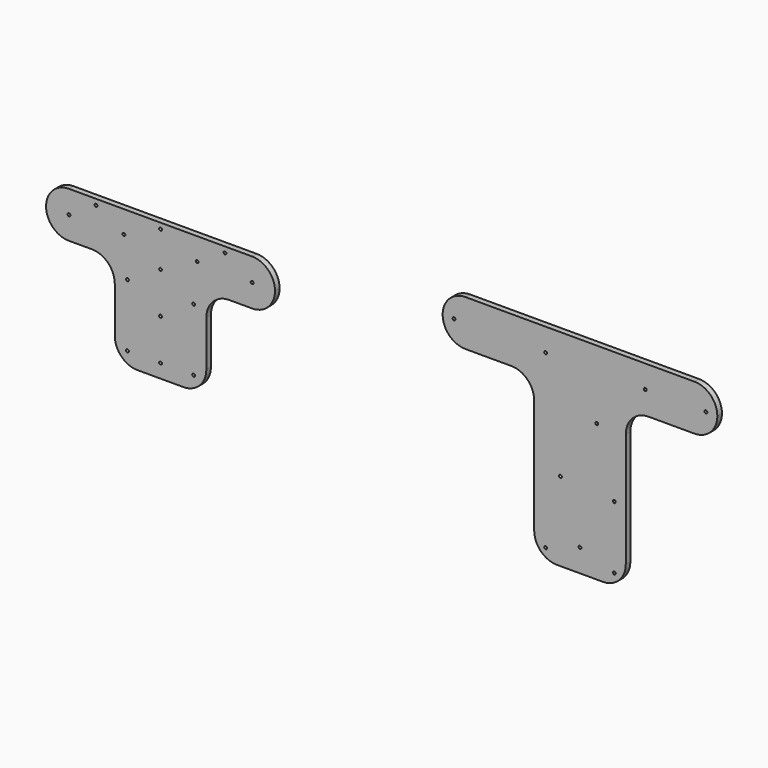
from build123d import *

# Parameters (mm, degrees)
F0_R     = 1.5875
F1_DEPTH = 6.35
F2_R     = 25.39999
F3_R     = 25.4
F4_R     = 25.39999
F5_R     = 1.5875
F6_DEPTH = 25.4


# Not quite as in the source:
# - a fillet or chamfer is up to 0.001 mm smaller than in the source, because OpenCascade refuses the exact size


with BuildPart() as f1:
    # F0 (on Front) → F1 (new body)
    with BuildSketch(Plane.XZ):
        Polygon((50.8, 114.3), (-50.8, 114.3), (-50.8, 63.5), (-50.8, -114.3), (-38.1, -114.3), (38.1, -114.3), (50.8, -114.3), (50.8, -31.75), (50.8, 63.5), (50.8, 88.9428858587), align=None)
        with BuildLine():
            ThreePointArc((-36.5125, -101.6), (-36.9774679849, -102.7225320151), (-38.1, -103.1875))
            ThreePointArc((-38.1, -103.1875), (-39.2225320151, -100.4774679849), (-36.5125, -101.6))
        make_face(mode=Mode.SUBTRACT)
        with BuildLine():
            ThreePointArc((39.6875, -101.6), (39.2225320151, -102.7225320151), (38.1, -103.1875))
            ThreePointArc((38.1, -103.1875), (36.9774679849, -100.4774679849), (39.6875, -101.6))
        make_face(mode=Mode.SUBTRACT)
        with Locations((0, -88.9)):
            Circle(F0_R, mode=Mode.SUBTRACT)
        with Locations((38.1, -31.75)):
            Circle(F0_R, mode=Mode.SUBTRACT)
        with Locations((-21.7083130796, -26.5298890234)):
            Circle(F0_R, mode=Mode.SUBTRACT)
        with Locations((18.6577301353, 38.1)):
            Circle(F0_R, mode=Mode.SUBTRACT)
        with Locations((-38.1000090512, 88.9428858587)):
            Circle(F0_R, mode=Mode.SUBTRACT)
        Polygon((-50.8, 63.5), (-50.8, 114.3), (-152.4, 114.3), (-152.4, 88.9), (-152.4, 63.5), align=None)
        with BuildLine():
            ThreePointArc((-138.1125, 88.9), (-139.7, 87.3125), (-141.2875, 88.9))
            ThreePointArc((-141.2875, 88.9), (-139.7, 90.4875), (-138.1125, 88.9))
        make_face(mode=Mode.SUBTRACT)
        with BuildLine():
            Line((72.3543986678, 114.3), (50.8, 114.3))
            Line((50.8, 114.3), (50.8, 88.9428858587))
            Line((50.8, 88.9428858587), (70.7668986678, 88.9428858587))
            ThreePointArc((70.7668986678, 88.9428858587), (71.2318666527, 90.0654178738), (72.3543986678, 90.5303858587))
            Line((72.3543986678, 90.5303858587), (72.3543986678, 114.3))
        make_face()
        with BuildLine():
            Line((70.7668986678, 88.9428858587), (50.8, 88.9428858587))
            Line((50.8, 88.9428858587), (50.8, 63.5))
            Line((50.8, 63.5), (152.4, 63.5))
            Line((152.4, 63.5), (152.4, 88.9))
            Line((152.4, 88.9), (152.4, 114.3))
            Line((152.4, 114.3), (72.3543986678, 114.3))
            Line((72.3543986678, 114.3), (72.3543986678, 90.5303858587))
            ThreePointArc((72.3543986678, 90.5303858587), (73.4769306829, 90.0654178738), (73.9418986678, 88.9428858587))
            ThreePointArc((73.9418986678, 88.9428858587), (72.3543986678, 87.3553858587), (70.7668986678, 88.9428858587))
        make_face()
        with Locations((139.7, 88.9)):
            Circle(F0_R, mode=Mode.SUBTRACT)
    extrude(amount=F1_DEPTH)

    # F2 (radius 25.4 in the source; OpenCascade refuses exactly that, so slightly less here)
    f2_edges = [f1.edges().sort_by_distance(p)[0] for p in [
        (-50.8, -3.175, 63.5),
        (50.8, -3.175, 63.5),
        (152.4, -3.175, 63.5),
        (152.4, -3.175, 114.3),
        (50.8, -3.175, -114.3),
        (-50.8, -3.175, -114.3),
        (-152.4, -3.175, 63.5),
        (-152.4, -3.175, 114.3),
    ]]
    fillet(f2_edges, radius=F2_R)


with BuildPart() as f1b:
    # F0 (on Front) → F1, piece 2 (new body)
    with BuildSketch(Plane.XZ):
        Polygon((-516.2082994461, 26.1577678084), (-516.2082994461, -75.4422321916), (-414.6082994461, -75.4422321916), (-414.6082994461, 26.1577678084), (-338.4082994461, 26.1577678084), (-338.4082994461, 76.9577678084), (-592.4082994461, 76.9577678084), (-592.4082994461, 26.1577678084), align=None)
        with Locations((-465.4082994461, -60.2022321916)):
            Circle(F0_R, mode=Mode.SUBTRACT)
    extrude(amount=F1_DEPTH)

    # F3
    f3_edges = [f1b.edges().sort_by_distance(p)[0] for p in [
        (-592.408299, -3.175, 26.157768),
        (-516.208299, -3.175, 26.157768),
        (-516.208299, -3.175, -75.442232),
        (-414.608299, -3.175, 26.157768),
        (-414.608299, -3.175, -75.442232),
        (-338.408299, -3.175, 76.957768),
    ]]
    fillet(f3_edges, radius=F3_R)

    # F4 (radius 25.4 in the source; OpenCascade refuses exactly that, so slightly less here)
    f4_edges = [f1b.edges().sort_by_distance(p)[0] for p in [
        (-338.408299, -3.175, 26.157768),
        (-592.408299, -3.175, 76.957768),
    ]]
    fillet(f4_edges, radius=F4_R)

    # F5 (on face) → F6 (cut)
    with BuildSketch(Plane.XZ.offset(6.35)):
        with Locations((-567.0082994461, 51.5577678084)):
            Circle(F5_R)
        with Locations((-363.8082994461, 104.2201220989)):
            Circle(F5_R)
        with Locations((-363.8082994461, 51.5577678084)):
            Circle(F5_R)
        with Locations((-506.0514450161, 52.1770399586)):
            Circle(F5_R)
        with Locations((-465.4082994461, 31.2377678084)):
            Circle(F5_R)
        with Locations((-465.4082994461, -14.4822321916)):
            Circle(F5_R)
        with Locations((-424.7651538761, 52.1770399586)):
            Circle(F5_R)
        with Locations((-502.1675247718, -60.2022321916)):
            Circle(F5_R)
        with Locations((-428.6490741204, -60.2022321916)):
            Circle(F5_R)
        with Locations((-428.6490741204, 9.309434332)):
            Circle(F5_R)
        with Locations((-502.1675247718, 9.309434332)):
            Circle(F5_R)
        with Locations((-465.4082994461, 70.6077678084)):
            Circle(F5_R)
        with Locations((-536.9790032417, 70.6077678084)):
            Circle(F5_R)
        with Locations((-393.8616867844, 70.6077678084)):
            Circle(F5_R)
    extrude(amount=-F6_DEPTH, mode=Mode.SUBTRACT)


solid = Compound([f1.part, f1b.part])
